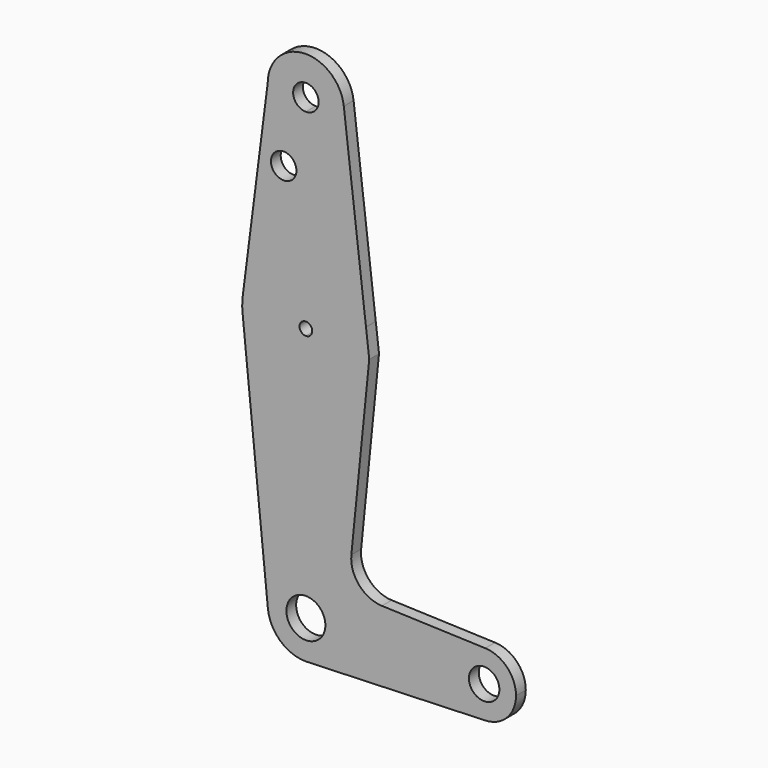
from build123d import *

# Parameters (mm, degrees)
F0_R     = 3.175
F1_DEPTH = 3.048


with BuildPart() as f1:
    # F0 (on Front) → F1 (new body)
    with BuildSketch(Plane.XZ):
        with BuildLine():
            ThreePointArc((-9.525, 114.3), (-6.7351920908, 107.5648079092), (0, 104.775))
            ThreePointArc((0, 104.775), (6.7351920908, 107.5648079092), (9.525, 114.3))
            ThreePointArc((9.525, 114.3), (9.5084619879, 114.8610486832), (9.4589053806, 115.4201490977))
            ThreePointArc((9.4589053806, 115.4201490977), (-0.5610486832, 123.8084619879), (-9.525, 114.3))
        make_face()
        with BuildLine():
            ThreePointArc((3.175, 114.3), (2.2450640303, 112.0549359697), (0, 111.125))
            ThreePointArc((0, 111.125), (-2.2450640303, 116.5450640303), (3.175, 114.3))
        make_face(mode=Mode.SUBTRACT)
        with BuildLine():
            ThreePointArc((9.525, 114.3), (6.7351920908, 107.5648079092), (0, 104.775))
            Line((0, 104.775), (0, 79.375))
            ThreePointArc((0, 79.375), (9.1908363712, 76.4438847259), (14.9877324754, 68.7329246359))
            Line((14.9877324754, 68.7329246359), (9.4589053806, 115.4201490977))
            ThreePointArc((9.4589053806, 115.4201490977), (9.5084619879, 114.8610486832), (9.525, 114.3))
        make_face()
        with BuildLine():
            Line((0, 79.375), (0, 104.775))
            ThreePointArc((0, 104.775), (-6.7351920908, 107.5648079092), (-9.525, 114.3))
            Line((-9.525, 114.3), (-15.7474569047, 65.5082893304))
            ThreePointArc((-15.7474569047, 65.5082893304), (-10.4912828548, 75.4142187767), (0, 79.375))
        make_face()
        with Locations((-5.5348160677, 97.4346920848)):
            Circle(F0_R, mode=Mode.SUBTRACT)
        with BuildLine():
            ThreePointArc((14.9877324754, 68.7329246359), (9.1908363712, 76.4438847259), (0, 79.375))
            Line((0, 79.375), (0, 65.0875))
            ThreePointArc((0, 65.0875), (1.1225320151, 64.6225320151), (1.5875, 63.5))
            ThreePointArc((1.5875, 63.5), (1.1225320151, 62.3774679849), (0, 61.9125))
            Line((0, 61.9125), (0, 47.625))
            ThreePointArc((0, 47.625), (10.6492737428, 51.7267849017), (15.7954255641, 61.9125))
            Line((15.7954255641, 61.9125), (14.9877324754, 68.7329246359))
        make_face()
        with BuildLine():
            Line((0, 65.0875), (0, 79.375))
            ThreePointArc((0, 79.375), (-10.4912828548, 75.4142187767), (-15.7474569047, 65.5082893304))
            ThreePointArc((-15.7474569047, 65.5082893304), (-15.8735876171, 63.7117573215), (-15.7954255641, 61.9125))
            ThreePointArc((-15.7954255641, 61.9125), (-10.6492737428, 51.7267849017), (0, 47.625))
            Line((0, 47.625), (0, 61.9125))
            ThreePointArc((0, 61.9125), (-1.5875, 63.5), (0, 65.0875))
        make_face()
        with BuildLine():
            Line((11.3408358685, 17.5898921545), (15.7954255641, 61.9125))
            ThreePointArc((15.7954255641, 61.9125), (10.6492737428, 51.7267849017), (0, 47.625))
            Line((0, 47.625), (0, 9.525))
            ThreePointArc((0, 9.525), (6.7351920908, 6.7351920908), (9.525, 0))
            Line((9.525, 0), (36.5125, 0))
            ThreePointArc((36.5125, 0), (38.9380895153, 5.7116327839), (44.7324052746, 7.9324746146))
            Line((44.7324052746, 7.9324746146), (18.968327868, 8.8497055806))
            ThreePointArc((18.968327868, 8.8497055806), (13.2612039825, 11.5674628959), (11.3408358685, 17.5898921545))
        make_face()
        with BuildLine():
            ThreePointArc((0, 47.625), (-10.6492737428, 51.7267849017), (-15.7954255641, 61.9125))
            Line((-15.7954255641, 61.9125), (-9.4772553384, -0.9525))
            ThreePointArc((-9.4772553384, -0.9525), (-7.063929059, 6.3895642457), (0, 9.525))
            Line((0, 9.525), (0, 47.625))
        make_face()
        with BuildLine():
            ThreePointArc((0, 9.525), (-7.063929059, 6.3895642457), (-9.4772553384, -0.9525))
            ThreePointArc((-9.4772553384, -0.9525), (-6.3895642457, -7.063929059), (0, -9.525))
            Line((0, -9.525), (0.6773435479, -9.500885786))
            ThreePointArc((0.6773435479, -9.500885786), (6.9705567315, -6.4912990883), (9.525, 0))
            Line((9.525, 0), (4.8608528189, 0))
            ThreePointArc((4.8608528189, 0), (-3.4371419906, -3.4371419906), (0, 4.8608528189))
            Line((0, 4.8608528189), (0, 9.525))
        make_face()
        with BuildLine():
            ThreePointArc((9.525, 0), (6.7351920908, 6.7351920908), (0, 9.525))
            Line((0, 9.525), (0, 4.8608528189))
            ThreePointArc((0, 4.8608528189), (3.4371419906, 3.4371419906), (4.8608528189, 0))
            Line((4.8608528189, 0), (9.525, 0))
        make_face()
        with BuildLine():
            Line((36.5125, 0), (9.525, 0))
            ThreePointArc((9.525, 0), (6.9705567315, -6.4912990883), (0.6773435479, -9.500885786))
            Line((0.6773435479, -9.500885786), (44.7324052746, -7.9324746146))
            ThreePointArc((44.7324052746, -7.9324746146), (38.9380895153, -5.7116327839), (36.5125, 0))
        make_face()
        with BuildLine():
            ThreePointArc((52.3875, 0), (50.1616327839, 5.5119104847), (44.7324052746, 7.9324746146))
            ThreePointArc((44.7324052746, 7.9324746146), (38.9380895153, 5.7116327839), (36.5125, 0))
            Line((36.5125, 0), (40.655729, 0))
            ThreePointArc((40.655729, 0), (44.45, 3.794271), (48.244271, 0))
            Line((48.244271, 0), (52.3875, 0))
        make_face()
        with BuildLine():
            Line((40.655729, 0), (36.5125, 0))
            ThreePointArc((36.5125, 0), (38.9380895153, -5.7116327839), (44.7324052746, -7.9324746146))
            ThreePointArc((44.7324052746, -7.9324746146), (50.1616327839, -5.5119104847), (52.3875, 0))
            Line((52.3875, 0), (48.244271, 0))
            ThreePointArc((48.244271, 0), (44.45, -3.794271), (40.655729, 0))
        make_face()
    extrude(amount=F1_DEPTH)


solid = f1.part
